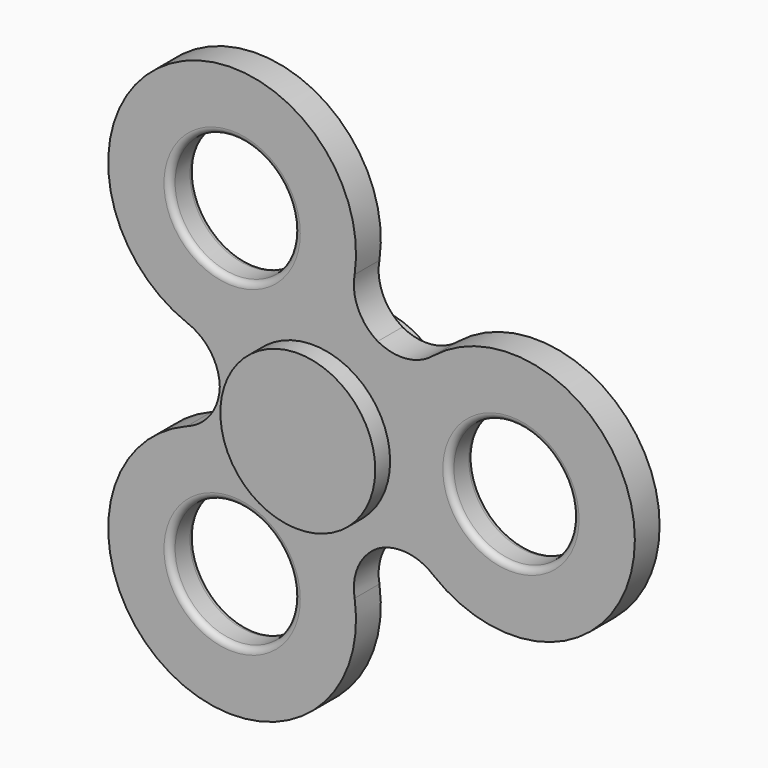
from build123d import *

# Parameters (mm, degrees)
F0_R      = 12.5
F1_DEPTH  = 3
F2_R      = 5
F2_R_2    = 4
F3_DEPTH  = 2
F4_R      = 3
F5_DEPTH  = 10
F7_R      = 6
F7_R_2    = 5
F8_DEPTH  = 10
F9_R      = 9
F9_R_2    = 8
F10_DEPTH = 10
F12_R     = 12.5
F13_DEPTH = 3
F14_R     = 4
F14_R_2   = 3
F15_DEPTH = 3
F17_R     = 10
F18_DEPTH = 2.5
F19_R     = 1
F20_COUNT = 3
F21_R     = 9
F22_DEPTH = 12.5


with BuildPart() as f1:
    # F0 (on Front) → F1 (new body)
    with BuildSketch(Plane.XZ):
        Circle(F0_R)
    extrude(amount=F1_DEPTH)

    # F2 (on face) → F3 (join)
    with BuildSketch(Plane.XZ.offset(3)):
        Circle(F2_R)
        Circle(F2_R_2, mode=Mode.SUBTRACT)
    extrude(amount=F3_DEPTH)

    # F4 (on face) → F5 (join)
    with BuildSketch(Plane.XZ.offset(3)):
        Circle(F4_R)
    extrude(amount=F5_DEPTH)

    # F12 (on offset) → F13 (join)
    with BuildSketch(Plane.XZ.offset(13)):
        Circle(F12_R)
    extrude(amount=F13_DEPTH)

    # F14 (on offset) → F15 (join)
    with BuildSketch(Plane.XZ.offset(13)):
        Circle(F14_R)
        Circle(F14_R_2, mode=Mode.SUBTRACT)
    extrude(amount=-F15_DEPTH)


with BuildPart() as f8:
    # F7 (on offset) → F8 (new body)
    with BuildSketch(Plane.XZ.offset(3)):
        Circle(F7_R)
        Circle(F7_R_2, mode=Mode.SUBTRACT)
    extrude(amount=F8_DEPTH)


with BuildPart() as f10:
    # F9 (on offset) → F10 (new body)
    with BuildSketch(Plane.XZ.offset(3)):
        Circle(F9_R)
        Circle(F9_R_2, mode=Mode.SUBTRACT)
    extrude(amount=F10_DEPTH)


with BuildPart() as f18:
    # F17 (on offset) → F18 (new body, symmetric)
    with BuildSketch(Plane.XZ.offset(8)):
        with BuildLine():
            Line((8.4944397181, 14.7128011735), (0, 0))
            Line((0, 0), (8.4944397181, -14.7128011735))
            ThreePointArc((8.4944397181, -14.7128011735), (13.1534822559, -13.7678782634), (17.5260798395, -15.6333398808))
            ThreePointArc((17.5260798395, -15.6333398808), (50, 0), (17.5260798395, 15.6333398808))
            ThreePointArc((17.5260798395, 15.6333398808), (13.1534822559, 13.7678782634), (8.4944397181, 14.7128011735))
        make_face()
        with Locations((30, 0)):
            Circle(F17_R, mode=Mode.SUBTRACT)
    extrude(amount=F18_DEPTH, both=True)

    # F19
    f19_edges = [f18.edges().sort_by_distance(p)[0] for p in [
        (20, -10.5, 0),
        (20, -5.5, 0),
    ]]
    fillet(f19_edges, radius=F19_R)

    # F20: F18 ×3 about axis
    f20_axis = Axis((0, -3, 0), (0, 1, 0))


with BuildPart() as f18_1:
    add(f18.part)
    for i in range(1, F20_COUNT):
        add(f18.part.rotate(f20_axis, i * 360 / F20_COUNT))

    # F21 (on offset) → F22 (cut, symmetric)
    with BuildSketch(Plane.XZ.offset(8)):
        Circle(F21_R)
    extrude(amount=F22_DEPTH, both=True, mode=Mode.SUBTRACT)


solid = Compound([f1.part, f8.part, f10.part, f18_1.part])
